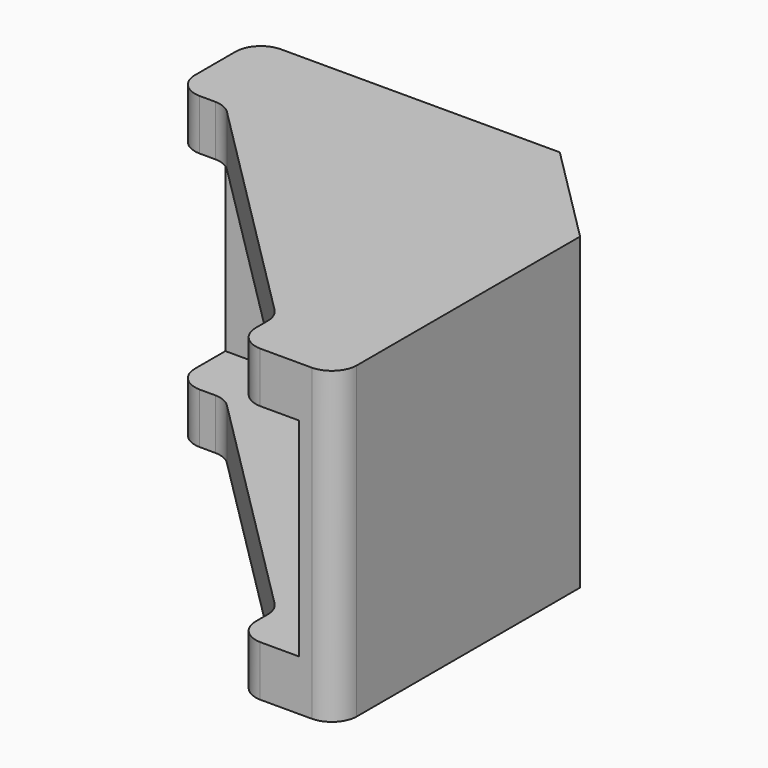
from build123d import *

# Parameters (mm, degrees)
F0_W        = 4
F0_H        = 12
F1_DEPTH    = 12.2
F2_W        = 2.5
F2_H        = 8.2
F3_DEPTH    = 14.5
F4_W        = 2.5
F4_H        = 8.2
F5_DEPTH    = 13.2
F6_SIZE     = 10
F7_R        = 2
F8_SIZE     = 4
F9_T1_DEPTH = 2
F9_T3_DEPTH = 2
F9_T5_DEPTH = 7.0048288267
F9_T7_DEPTH = 17.2048288267
F9_T9_DEPTH = 7.0048288267


# Not quite as in the source:
# - a fillet or chamfer that OpenCascade refuses, or shapes differently, is made with other operations: its cross-section is extruded or revolved along the edge and cut away or added


with BuildPart() as f1:
    # F0 (on Top) → F1 (new body)
    with BuildSketch(Plane.XY):
        Polygon((-29.984754981, 31.7928069385), (-45.984754981, 31.7928069385), (-45.984754981, 27.7928069385), (-33.984754981, 27.7928069385), (-29.984754981, 27.7928069385), align=None)
        with Locations((-31.984754981, 21.7928069385)):
            Rectangle(F0_W, F0_H)
    extrude(amount=F1_DEPTH)

    # F2 (on face) → F3 (cut)
    with BuildSketch(Plane(origin=(-45.984754981, 0, 0), x_dir=(0, -1, 0), z_dir=(-1, 0, 0))):
        with Locations((-29.0428069385, 6.1)):
            Rectangle(F2_W, F2_H)
    extrude(amount=-F3_DEPTH, mode=Mode.SUBTRACT)

    # F4 (on face) → F5 (cut)
    with BuildSketch(Plane.XZ.offset(-15.7928069385)):
        with Locations((-32.734754981, 6.1)):
            Rectangle(F4_W, F4_H)
    extrude(amount=-F5_DEPTH, mode=Mode.SUBTRACT)

    # F6
    f6_edges = [f1.edges().sort_by_distance(p)[0] for p in [
        (-33.984755, 27.792807, 1),
        (-33.984755, 27.792807, 11.2),
    ]]
    chamfer(f6_edges, length=F6_SIZE)

    # F7
    f7_edges = [f1.edges().sort_by_distance(p)[0] for p in [
        (-31.484755, 30.292807, 6.1),
    ]]
    fillet(f7_edges, radius=F7_R)

    # F8
    f8_edges = [f1.edges().sort_by_distance(p)[0] for p in [
        (-29.984755, 31.792807, 6.1),
    ]]
    chamfer(f8_edges, length=F8_SIZE)

    # F9: fillet of radius 1 on 14 edges, made by hand

    # F9_s2 → F9_t1 (join)
    with BuildSketch(Plane.XY):
        with BuildLine():
            ThreePointArc((-44.3997969705, 27.7932069385), (-44.0161950979, 27.7169037819), (-43.690993133, 27.4996107759))
            Line((-43.690993133, 27.4996107759), (-43.6201127493, 27.5704911597))
            ThreePointArc((-43.6201127493, 27.5704911597), (-43.7671350946, 27.7169478196), (-43.9138745973, 27.8636873222))
            Line((-43.9138745973, 27.8636873222), (-43.984754981, 27.8930469385))
            ThreePointArc((-43.984754981, 27.8930469385), (-44.1922759758, 27.8930469385), (-44.3997969705, 27.8934469385))
            Line((-44.3997969705, 27.8934469385), (-44.3997969705, 27.7932069385))
        make_face()
        with BuildLine():
            ThreePointArc((-34.2779511435, 18.0865687864), (-34.0606581376, 17.7613668216), (-33.984354981, 17.377764949))
            Line((-33.984354981, 17.377764949), (-33.884114981, 17.377764949))
            ThreePointArc((-33.884114981, 17.377764949), (-33.884514981, 17.5852859437), (-33.884514981, 17.7928069385))
            Line((-33.884514981, 17.7928069385), (-33.9138745973, 17.8636873222))
            ThreePointArc((-33.9138745973, 17.8636873222), (-34.0606140999, 18.0104268249), (-34.2070707598, 18.1574491702))
            Line((-34.2070707598, 18.1574491702), (-34.2779511435, 18.0865687864))
        make_face()
    extrude(amount=F9_T1_DEPTH)

    # F9_s4 → F9_t3 (join)
    with BuildSketch(Plane.XY.offset(10.2)):
        with BuildLine():
            ThreePointArc((-44.3997969705, 27.7932069385), (-44.0161950979, 27.7169037819), (-43.690993133, 27.4996107759))
            Line((-43.690993133, 27.4996107759), (-43.6201127493, 27.5704911597))
            ThreePointArc((-43.6201127493, 27.5704911597), (-43.7671350946, 27.7169478196), (-43.9138745973, 27.8636873222))
            Line((-43.9138745973, 27.8636873222), (-43.984754981, 27.8930469385))
            ThreePointArc((-43.984754981, 27.8930469385), (-44.1922759758, 27.8930469385), (-44.3997969705, 27.8934469385))
            Line((-44.3997969705, 27.8934469385), (-44.3997969705, 27.7932069385))
        make_face()
        with BuildLine():
            ThreePointArc((-33.984354981, 17.377764949), (-34.0606581376, 17.7613668216), (-34.2779511435, 18.0865687864))
            Line((-34.2779511435, 18.0865687864), (-34.2070707598, 18.1574491702))
            ThreePointArc((-34.2070707598, 18.1574491702), (-34.0606140999, 18.0104268249), (-33.9138745973, 17.8636873222))
            Line((-33.9138745973, 17.8636873222), (-33.884514981, 17.7928069385))
            ThreePointArc((-33.884514981, 17.7928069385), (-33.884514981, 17.5852859437), (-33.884114981, 17.377764949))
            Line((-33.884114981, 17.377764949), (-33.984354981, 17.377764949))
        make_face()
    extrude(amount=F9_T3_DEPTH)

    # F9_s6 → F9_t5 (cut)
    with BuildSketch(Plane.XY.offset(7.6975855866)):
        with BuildLine():
            ThreePointArc((-45.985154981, 28.7937726239), (-45.6918617622, 28.0857001573), (-44.9837892956, 27.7924069385))
            Line((-44.9837892956, 27.7924069385), (-44.9837892956, 27.6922703699))
            ThreePointArc((-44.9837892956, 27.6922703699), (-45.4842721383, 27.6926703699), (-45.984754981, 27.6926703699))
            Line((-45.984754981, 27.6926703699), (-46.0848915495, 27.7928069385))
            ThreePointArc((-46.0848915495, 27.7928069385), (-46.0848915495, 28.2932897812), (-46.0852915495, 28.7937726239))
            Line((-46.0852915495, 28.7937726239), (-45.985154981, 28.7937726239))
        make_face()
        with BuildLine():
            ThreePointArc((-32.9837892956, 15.7924069385), (-33.6918617622, 16.0857001573), (-33.985154981, 16.7937726239))
            Line((-33.985154981, 16.7937726239), (-34.0852915495, 16.7937726239))
            ThreePointArc((-34.0852915495, 16.7937726239), (-34.0848915495, 16.2932897812), (-34.0848915495, 15.7928069385))
            Line((-34.0848915495, 15.7928069385), (-33.984754981, 15.6926703699))
            ThreePointArc((-33.984754981, 15.6926703699), (-33.4842721383, 15.6926703699), (-32.9837892956, 15.6922703699))
            Line((-32.9837892956, 15.6922703699), (-32.9837892956, 15.7924069385))
        make_face()
    extrude(amount=F9_T5_DEPTH, mode=Mode.SUBTRACT)

    # F9_s8 → F9_t7 (cut)
    with BuildSketch(Plane.XY.offset(-2.5024144134)):
        with BuildLine():
            ThreePointArc((-29.984354981, 16.7937726239), (-30.2776481998, 16.0857001573), (-30.9857206664, 15.7924069385))
            Line((-30.9857206664, 15.7924069385), (-30.9857206664, 15.6922703699))
            ThreePointArc((-30.9857206664, 15.6922703699), (-30.4852378237, 15.6926703699), (-29.984754981, 15.6926703699))
            Line((-29.984754981, 15.6926703699), (-29.8846184125, 15.7928069385))
            ThreePointArc((-29.8846184125, 15.7928069385), (-29.8846184125, 16.2932897812), (-29.8842184125, 16.7937726239))
            Line((-29.8842184125, 16.7937726239), (-29.984354981, 16.7937726239))
        make_face()
        with BuildLine():
            ThreePointArc((-45.985154981, 30.7918412531), (-45.6918617622, 31.4999137197), (-44.9837892956, 31.7932069385))
            Line((-44.9837892956, 31.7932069385), (-44.9837892956, 31.893343507))
            ThreePointArc((-44.9837892956, 31.893343507), (-45.4842721383, 31.892943507), (-45.984754981, 31.892943507))
            Line((-45.984754981, 31.892943507), (-46.0848915495, 31.7928069385))
            ThreePointArc((-46.0848915495, 31.7928069385), (-46.0848915495, 31.2923240958), (-46.0852915495, 30.7918412531))
            Line((-46.0852915495, 30.7918412531), (-45.985154981, 30.7918412531))
        make_face()
    extrude(amount=F9_T7_DEPTH, mode=Mode.SUBTRACT)

    # F9_s10 → F9_t9 (cut)
    with BuildSketch(Plane.XY.offset(-2.5024144134)):
        with BuildLine():
            ThreePointArc((-32.9837892956, 15.7924069385), (-33.6918617622, 16.0857001573), (-33.985154981, 16.7937726239))
            Line((-33.985154981, 16.7937726239), (-34.0852915495, 16.7937726239))
            ThreePointArc((-34.0852915495, 16.7937726239), (-34.0848915495, 16.2932897812), (-34.0848915495, 15.7928069385))
            Line((-34.0848915495, 15.7928069385), (-33.984754981, 15.6926703699))
            ThreePointArc((-33.984754981, 15.6926703699), (-33.4842721383, 15.6926703699), (-32.9837892956, 15.6922703699))
            Line((-32.9837892956, 15.6922703699), (-32.9837892956, 15.7924069385))
        make_face()
        with BuildLine():
            ThreePointArc((-44.9837892956, 27.7924069385), (-45.6918617622, 28.0857001573), (-45.985154981, 28.7937726239))
            Line((-45.985154981, 28.7937726239), (-46.0852915495, 28.7937726239))
            ThreePointArc((-46.0852915495, 28.7937726239), (-46.0848915495, 28.2932897812), (-46.0848915495, 27.7928069385))
            Line((-46.0848915495, 27.7928069385), (-45.984754981, 27.6926703699))
            ThreePointArc((-45.984754981, 27.6926703699), (-45.4842721383, 27.6926703699), (-44.9837892956, 27.6922703699))
            Line((-44.9837892956, 27.6922703699), (-44.9837892956, 27.7924069385))
        make_face()
    extrude(amount=F9_T9_DEPTH, mode=Mode.SUBTRACT)


solid = f1.part
